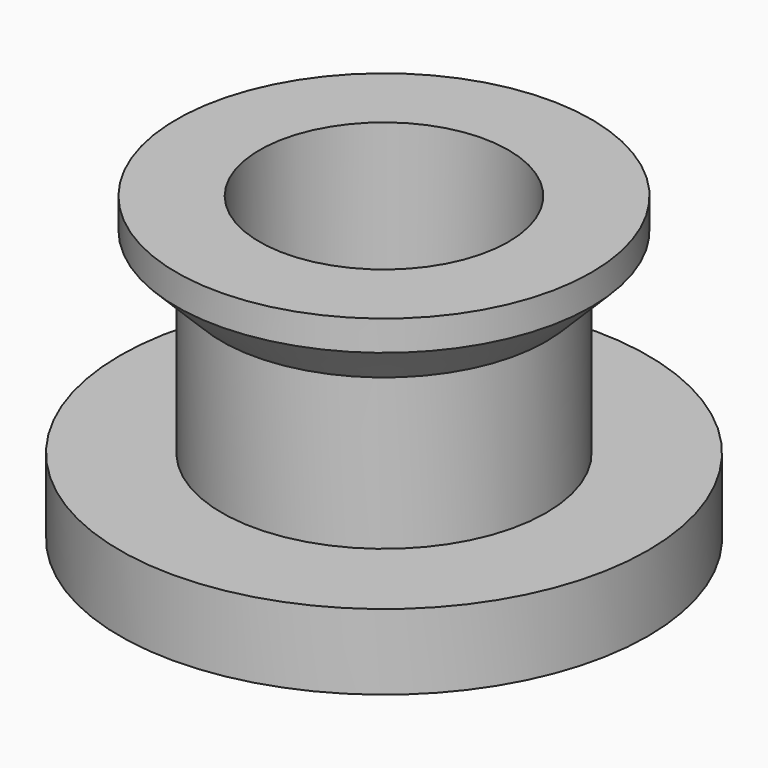
from build123d import *

# Parameters (mm, degrees)
F0_R     = 3.5
F0_R_2   = 2.15
F0_R_3   = 1.65
F1_DEPTH = 1
F2_R     = 2.15
F2_R_2   = 1.65
F3_DEPTH = 2
F4_R     = 2.75
F4_R_2   = 2.15
F4_R_3   = 1.65
F5_DEPTH = 1
F6_SIZE  = 0.59999


# Not quite as in the source:
# - a fillet or chamfer is up to 0.001 mm smaller than in the source, because OpenCascade refuses the exact size


with BuildPart() as f1:
    # F0 (on Top) → F1 (new body)
    with BuildSketch(Plane.XY):
        Circle(F0_R)
        Circle(F0_R_2, mode=Mode.SUBTRACT)
        Circle(F0_R_2)
        Circle(F0_R_3, mode=Mode.SUBTRACT)
    extrude(amount=F1_DEPTH)

    # F2 (on face) → F3 (join)
    with BuildSketch(Plane.XY.offset(1)):
        Circle(F2_R)
        Circle(F2_R_2, mode=Mode.SUBTRACT)
    extrude(amount=F3_DEPTH)

    # F4 (on face) → F5 (join)
    with BuildSketch(Plane.XY.offset(3)):
        Circle(F4_R)
        Circle(F4_R_2, mode=Mode.SUBTRACT)
        Circle(F4_R_2)
        Circle(F4_R_3, mode=Mode.SUBTRACT)
    extrude(amount=F5_DEPTH)

    # F6 (size 0.6 in the source; OpenCascade refuses exactly that, so slightly less here)
    f6_edges = [f1.edges().sort_by_distance(p)[0] for p in [
        (-2.75, 0, 3),
    ]]
    chamfer(f6_edges, length=F6_SIZE)


solid = f1.part
